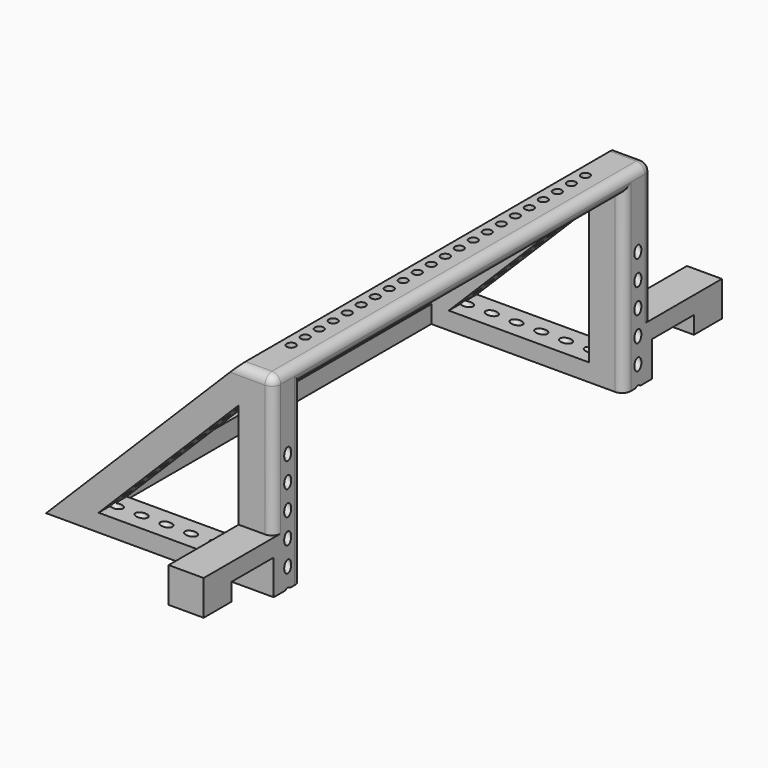
from build123d import *

# Parameters (mm, degrees)
F1_DEPTH  = 10
F3_DEPTH  = 20
F4_W      = 10
F4_H      = 10
F5_DEPTH  = 20
F6_W      = 10
F6_H      = 10
F7_DEPTH  = 20
F8_W      = 10
F8_H      = 10
F9_DEPTH  = 20
F11_DEPTH = 10
F13_DEPTH = 20
F14_DEPTH = 20
F15_DEPTH = 10
F17_DEPTH = 20
F18_DEPTH = 10
F20_R     = 4.99999
F22_D     = 5
F23_DEPTH = 250
F25_D     = 5
F27_D     = 5


# Not quite as in the source:
# - a fillet or chamfer is up to 0.001 mm smaller than in the source, because OpenCascade refuses the exact size
# - a pattern or mirror of a feature is missing from the dataset's text; its kind, count and spacing are read off the source's solid


with BuildPart() as f1:
    # F0 (on Right) → F1 (new body)
    with BuildSketch(Plane.YZ):
        Polygon((0, -100), (0, 0), (250, 0), (250, -100), (260, -100), (260, 10), (-10, 10), (-10, -100), align=None)
    extrude(amount=F1_DEPTH)

    # F2 (on face) → F3 (join)
    with BuildSketch(Plane.YZ.offset(10)):
        Polygon((-40, -80), (-10, -80), (-10, -70), (-60, -70), (-60, -90), (-40, -90), align=None)
        Polygon((310, -70), (260, -70), (260, -80), (290, -80), (290, -90), (310, -90), align=None)
    extrude(amount=-F3_DEPTH)

    # F4 (on face) → F5 (join)
    with BuildSketch(Plane.YZ.offset(10)):
        with Locations((-5, -75)):
            Rectangle(F4_W, F4_H)
        with Locations((255, -75)):
            Rectangle(F4_W, F4_H)
    extrude(amount=-F5_DEPTH)

    # F6 (on face) → F7 (join)
    with BuildSketch(Plane(origin=(0, 0, -80), x_dir=(1, 0, 0), z_dir=(0, 0, -1))):
        with Locations((-5, -255)):
            Rectangle(F6_W, F6_H)
    extrude(amount=F7_DEPTH)

    # F8 (on face) → F9 (join)
    with BuildSketch(Plane(origin=(0, 0, -80), x_dir=(1, 0, 0), z_dir=(0, 0, -1))):
        with Locations((-5, 5)):
            Rectangle(F8_W, F8_H)
    extrude(amount=F9_DEPTH)

    # F10 (on face) → F11 (join)
    with BuildSketch(Plane(origin=(0, 0, 0), x_dir=(0, -1, 0), z_dir=(-1, 0, 0))):
        Polygon((10, 10), (-260, 10), (-260, -70), (-250, -70), (-250, 0), (0, 0), (0, -70), (10, -70), align=None)
    extrude(amount=F11_DEPTH)

    # F12 (on face) → F13 (join)
    with BuildSketch(Plane.XZ.offset(10)):
        Polygon((-10, 0), (-10, 10), (-110, -90), (-100, -90), align=None)
        Polygon((-10, -90), (-90, -90), (-100, -100), (-10, -100), align=None)
        Polygon((-100, -90), (-110, -90), (-110, -100), align=None)
        Polygon((-110, -100), (-110, -90), (-120, -100), align=None)
    extrude(amount=-F13_DEPTH)

    # F12 (on face) → F14 (join)
    with BuildSketch(Plane.XZ.offset(10)):
        Polygon((10, 10), (-10, 10), (-10, 0), (-10, -10), (-10, -70), (10, -70), align=None)
        Polygon((-90, -90), (-100, -90), (-110, -100), (-100, -100), align=None)
    extrude(amount=-F14_DEPTH)

    # F15 (add): a face of the model
    f15_faces = [f1.faces().sort_by_distance(p)[0] for p in [
        (0, 0, -85),
    ]]
    extrude(f15_faces, amount=F15_DEPTH)

    # F16 (on face) → F17 (join)
    with BuildSketch(Plane(origin=(0, 260, 0), x_dir=(-1, 0, 0), z_dir=(0, 1, 0))):
        Polygon((110, -90), (10, 10), (10, -10), (90, -90), align=None)
        Polygon((120, -100), (110, -90), (90, -90), (10, -90), (10, -100), align=None)
    f17 = extrude(amount=-F17_DEPTH)

    # F17_copies: F17 across plane
    add(f17.mirror(Plane(origin=(0, 125, 0), x_dir=(0, 0, -1), z_dir=(0, -1, 0))))

    # F18 (add): a face of the model
    f18_faces = [f1.faces().sort_by_distance(p)[0] for p in [
        (0, 250, -50),
    ]]
    extrude(f18_faces, amount=F18_DEPTH)

    # F20 (radius 5 in the source; OpenCascade refuses exactly that, so slightly less here)
    f20_edges = [f1.edges().sort_by_distance(p)[0] for p in [
        (10, 125, 10),
        (10, 125, 0),
        (10, 10, -50),
        (10, 240, -50),
        (10, -10, -30),
        (10, 260, -30),
        (0, 260, 10),
        (0, -10, 10),
    ]]
    fillet(f20_edges, radius=F20_R)

    # F22 (through all)
    with Locations(Plane.XY.offset(10)):
        with Locations((-4, 20), (-4, 30), (-4, 40), (-4, 50), (-4, 60), (-4, 70), (-4, 80), (-4, 90), (-4, 100), (-4, 110), (-4, 120), (-4, 130), (-4, 140), (-4, 150), (-4, 140), (-4, 160), (-4, 170), (-4, 180), (-4, 200), (-4, 210), (-4, 220), (-4, 230), (-4, 190)):
            Hole(F22_D / 2)

    # F19 (on face) → F23 (join)
    with BuildSketch(Plane.XZ.offset(-240)):
        Polygon((-100, -100), (-100, -90), (-110, -90), (-120, -100), align=None)
    extrude(amount=F23_DEPTH)

    # F25 (through all)
    with Locations(Plane.XY.offset(-90)):
        with Locations((-105, 20), (-105, 30), (-105, 40), (-105, 50), (-105, 60), (-105, 70), (-105, 80), (-105, 90), (-105, 100), (-105, 110), (-105, 120), (-105, 130), (-105, 140), (-105, 150), (-105, 160), (-105, 170), (-105, 180), (-105, 190), (-105, 200), (-105, 210), (-105, 220), (-105, 230)):
            Hole(F25_D / 2)

    # F27 (through all)
    with Locations(Plane(origin=(-10, 0, 10), x_dir=(0, -1, 0), z_dir=(-0.7071067812, 0, 0.7071067812))):
        with Locations((0, -15.563491861), (0, -25.563491861), (0, -35.563491861), (0, -45.563491861), (0, -55.563491861), (0, -65.563491861), (0, -75.563491861), (0, -85.563491861), (0, -95.563491861), (0, -105.563491861), (0, -115.563491861), (0, -125.563491861), (-250, -15.563491861), (-250, -25.563491861), (-250, -35.563491861), (-250, -45.563491861), (-250, -55.563491861), (-250, -65.563491861), (-250, -75.563491861), (-250, -85.563491861), (-250, -95.563491861), (-250, -105.563491861), (-250, -115.563491861), (-250, -125.563491861)):
            Hole(F27_D / 2)


solid = f1.part
